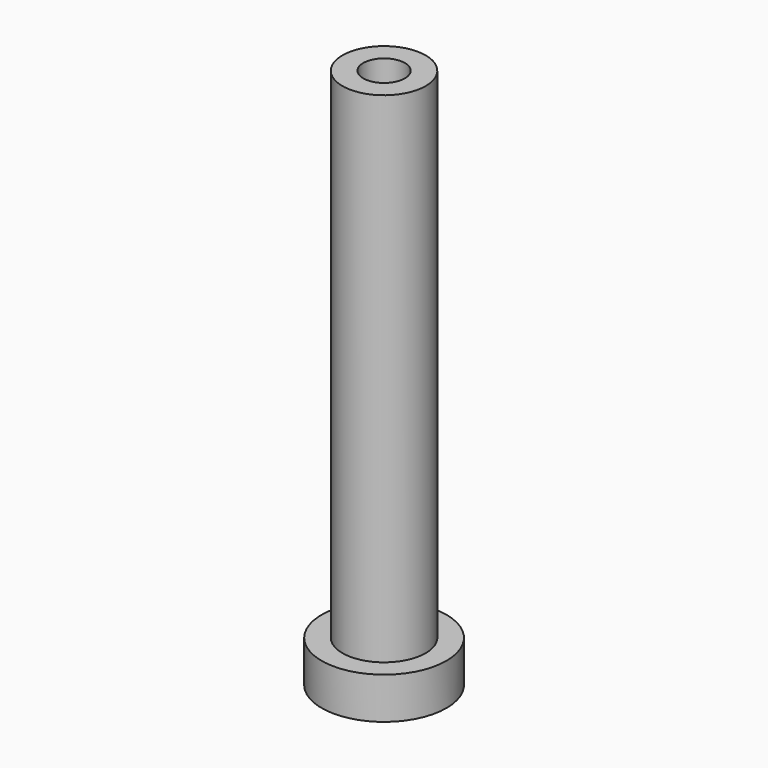
from build123d import *

# Parameters (mm, degrees)
F0_R     = 5
F1_DEPTH = 60
F2_R     = 7.5
F2_R_2   = 5
F3_DEPTH = 5
F4_R     = 2.5
F5_DEPTH = 25


with BuildPart() as f1:
    # F0 (on Top) → F1 (new body)
    with BuildSketch(Plane.XY):
        Circle(F0_R)
    extrude(amount=F1_DEPTH)

    # F2 (on face) → F3 (join)
    with BuildSketch(Plane(origin=(0, 0, 0), x_dir=(1, 0, 0), z_dir=(0, 0, -1))):
        Circle(F2_R)
        Circle(F2_R_2, mode=Mode.SUBTRACT)
        Circle(F2_R_2)
    extrude(amount=F3_DEPTH)

    # F4 (on face) → F5 (cut)
    with BuildSketch(Plane.XY.offset(60)):
        Circle(F4_R)
    extrude(amount=-F5_DEPTH, mode=Mode.SUBTRACT)


solid = f1.part
